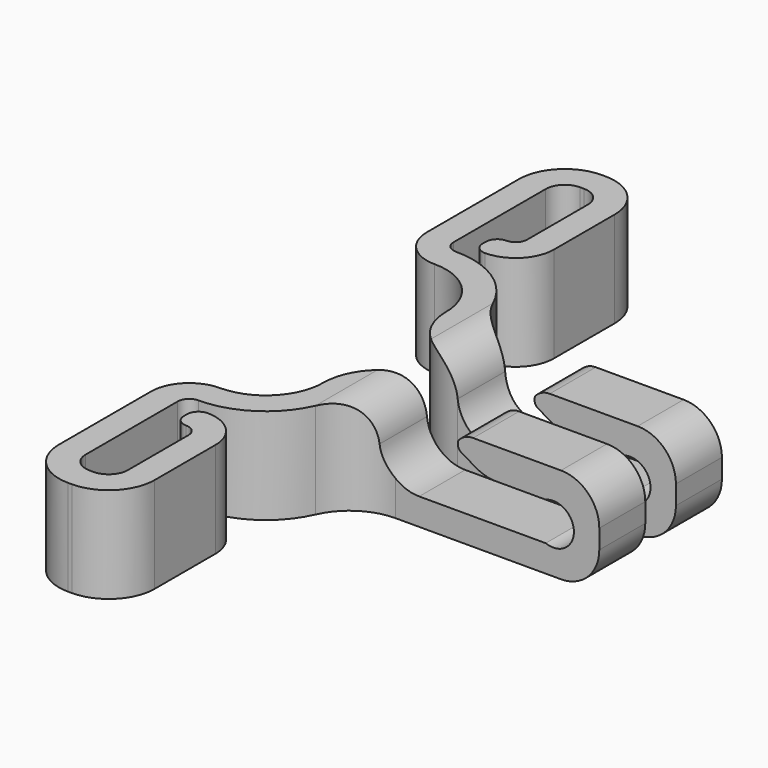
from build123d import *

# Parameters (mm, degrees)
F1_DEPTH    = 25
F3_DEPTH    = 82.001
F4_R        = 5.375
F5_DEPTH    = 82.001
F6_T1_DEPTH = 64.9941188264
F6_T3_DEPTH = 65
F7_T1_DEPTH = 28.821565156


# Not quite as in the source:
# - a fillet or chamfer that OpenCascade refuses, or shapes differently, is made with other operations: its cross-section is extruded or revolved along the edge and cut away or added


with BuildPart() as f1:
    # F0 (on Top) → F1 (new body)
    with BuildSketch(Plane.XY):
        with BuildLine():
            Line((-25, 70), (-25, 40))
            ThreePointArc((-25, 40), (-22.0710678119, 32.9289321881), (-15, 30))
            ThreePointArc((-15, 30), (-4.3933982822, 25.6066017178), (0, 15))
            ThreePointArc((0, 15), (4.3933982822, 4.3933982822), (15, 0))
            Line((15, 0), (72, 0))
            Line((72, 0), (72, 15))
            Line((72, 15), (18.8230690506, 15))
            ThreePointArc((18.8230690506, 15), (10.6443226985, 17.4258953357), (5.1110140301, 23.9189189189))
            ThreePointArc((5.1110140301, 23.9189189189), (-3.0045053503, 33.4420201743), (-15, 37))
            ThreePointArc((-15, 37), (-17.1213203436, 37.8786796564), (-18, 40))
            Line((-18, 40), (-18, 70))
            ThreePointArc((-18, 70), (-16.5355339059, 73.5355339059), (-13, 75))
            Line((-13, 75), (-12, 75))
            ThreePointArc((-12, 75), (-8.4644660941, 73.5355339059), (-7, 70))
            Line((-7, 70), (-7, 50.2319021523))
            ThreePointArc((-7, 50.2319021523), (-7.8786796564, 48.1105818087), (-10, 47.2319021523))
            ThreePointArc((-10, 47.2319021523), (-12.1213203436, 46.3532224959), (-13, 44.2319021523))
            Line((-13, 44.2319021523), (-13, 43.2319021523))
            ThreePointArc((-13, 43.2319021523), (-12.1213203436, 41.1105818087), (-10, 40.2319021523))
            ThreePointArc((-10, 40.2319021523), (-2.9289321881, 43.1608343404), (0, 50.2319021523))
            Line((0, 50.2319021523), (0, 70))
            ThreePointArc((0, 70), (-3.5147186258, 78.4852813742), (-12, 82))
            Line((-12, 82), (-13, 82))
            ThreePointArc((-13, 82), (-21.4852813742, 78.4852813742), (-25, 70))
        make_face()
    extrude(amount=F1_DEPTH)

    # F2 (on face) → F3 (cut, through all)
    with BuildSketch(Plane.XZ):
        with BuildLine():
            Line((40, 31.3886217773), (15, 31.3886217773))
            Line((15, 31.3886217773), (15, 17))
            ThreePointArc((15, 17), (17.9289321881, 9.9289321881), (25, 7))
            Line((25, 7), (60, 7))
            ThreePointArc((60, 7), (63.5355339059, 8.4644660941), (65, 12))
            ThreePointArc((65, 12), (63.5355339059, 15.5355339059), (60, 17))
            Line((60, 17), (45, 17))
            ThreePointArc((45, 17), (42.411809549, 17.3407417371), (40, 18.3397459622))
            Line((40, 18.3397459622), (36.0817218342, 20.6019649159))
            ThreePointArc((36.0817218342, 20.6019649159), (35.1498701816, 21.8163776333), (35.3496710266, 23.3340157235))
            Line((35.3496710266, 23.3340157235), (40, 31.3886217773))
        make_face()
    extrude(amount=-F3_DEPTH, mode=Mode.SUBTRACT)

    # F4 (on face) → F5 (cut, through all)
    with BuildSketch(Plane.XZ):
        with Locations((60, 12)):
            Circle(F4_R)
    extrude(amount=-F5_DEPTH, mode=Mode.SUBTRACT)

    # F6: fillet of radius 10 on 3 edges, made by hand

    # F6_s2 → F6_t1 (cut)
    with BuildSketch(Plane.XZ.offset(-40.244746971)):
        with BuildLine():
            ThreePointArc((5.1002512579, 25), (11.8084551904, 22.4161984871), (15.0501256289, 16))
            Line((15.0501256289, 16), (16.045113066, 16.1))
            ThreePointArc((16.045113066, 16.1), (16, 17), (16, 25))
            Line((16, 25), (15, 26))
            Line((15, 26), (5.1002512579, 26))
            Line((5.1002512579, 26), (5.1002512579, 25))
        make_face()
    extrude(amount=F6_T1_DEPTH, mode=Mode.SUBTRACT)

    # F6_s4 → F6_t3 (cut)
    with BuildSketch(Plane.XZ.offset(-40)):
        with BuildLine():
            ThreePointArc((72, 15), (69.0710678119, 22.0710678119), (62, 25))
            Line((62, 25), (72, 25))
            Line((72, 25), (72, 15))
        make_face()
        with BuildLine():
            ThreePointArc((72, 10), (69.0710678119, 2.9289321881), (62, 0))
            Line((62, 0), (72, 0))
            Line((72, 0), (72, 10))
        make_face()
    extrude(amount=F6_T3_DEPTH, mode=Mode.SUBTRACT)

    # F7: fillet of radius 5 on 1 edges, made by hand

    # F7_s2 → F7_t1 (cut)
    with BuildSketch(Plane.XZ.offset(-21.910782578)):
        with BuildLine():
            ThreePointArc((35.3496710266, 23.3340157235), (37.0350169957, 24.5645415223), (39.0758405283, 25))
            Line((39.0758405283, 25), (39.0758405283, 25.1))
            Line((39.0758405283, 25.1), (36.3115274971, 25.1))
            Line((36.3115274971, 25.1), (36.2249249567, 25.05))
            ThreePointArc((36.2249249567, 25.05), (35.7439967215, 24.2170078618), (35.2751476366, 23.400696038))
            Line((35.2751476366, 23.400696038), (35.3496710266, 23.3340157235))
        make_face()
    extrude(amount=F7_T1_DEPTH, mode=Mode.SUBTRACT)


with BuildPart() as f9_1:
    # F9: instance of F1
    add(f1.part.mirror(Plane(origin=(47.9199972847, -5, 10.7001036471), x_dir=(1, 0, 0), z_dir=(0, -1, 0))))


solid = Compound([f1.part, f9_1.part])
